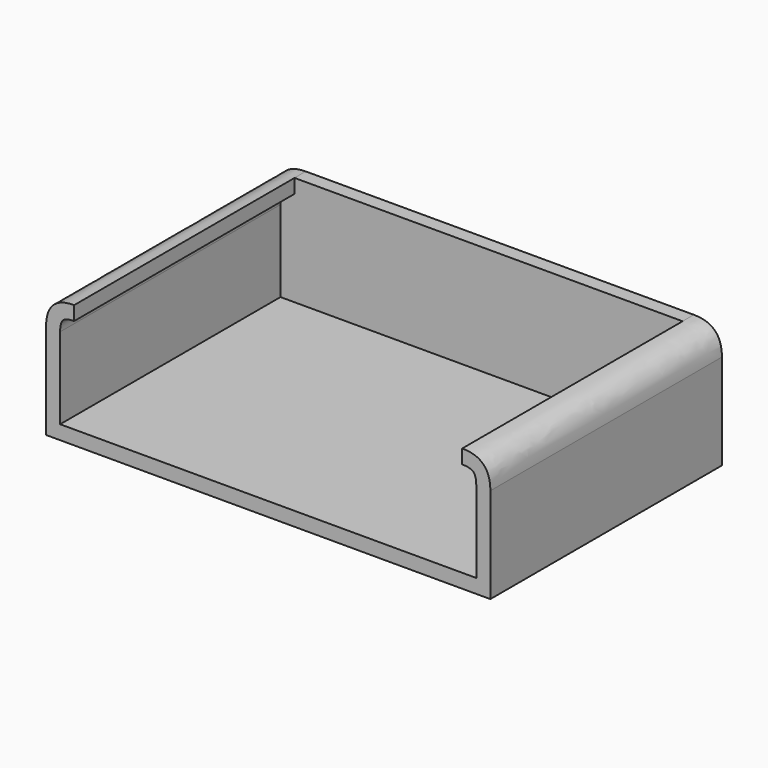
from build123d import *

# Parameters (mm, degrees)
F0_W        = 79.0347680449
F0_H        = 51.5021067113
F1_DEPTH    = 21.9734124839
F2_T1_DEPTH = 76.5021067113
F3_T        = 2.5


# Not quite as in the source:
# - a fillet or chamfer that OpenCascade refuses, or shapes differently, is made with other operations: its cross-section is extruded or revolved along the edge and cut away or added
# - a shell that OpenCascade refuses in one call is made with other operations: the cavity is built on its own and cut out


with BuildPart() as f1:
    # F0 (on Top) → F1 (new body)
    with BuildSketch(Plane.XY):
        with Locations((-4.2740143836, 13.997332193)):
            Rectangle(F0_W, F0_H)
    extrude(amount=F1_DEPTH)

    # F2: fillet of radius 5 on 2 edges, made by hand

    # F2_s2 → F2_t1 (cut)
    with BuildSketch(Plane.XZ.offset(-52.2483855486)):
        with BuildLine():
            add(Edge.make_bspline(
                [(-43.791398406, 16.9734124839), (-43.791398406, 21.9734124839), (-38.791398406, 21.9734124839)],
                knots=[0, 0, 0, 1, 1, 1], degree=2, weights=[1, 1, 1]))
            Line((-38.791398406, 21.9734124839), (-43.791398406, 21.9734124839))
            Line((-43.791398406, 21.9734124839), (-43.791398406, 16.9734124839))
        make_face()
        with BuildLine():
            add(Edge.make_bspline(
                [(35.2433696389, 16.9734124839), (35.2433696389, 21.9734124839), (30.2433696389, 21.9734124839)],
                knots=[0, 0, 0, 1, 1, 1], degree=2, weights=[1, 1, 1]))
            Line((30.2433696389, 21.9734124839), (35.2433696389, 21.9734124839))
            Line((35.2433696389, 21.9734124839), (35.2433696389, 16.9734124839))
        make_face()
    extrude(amount=F2_T1_DEPTH, mode=Mode.SUBTRACT)

    # F3: shell of thickness 2.5, made by hand


with BuildPart() as f3_core1:
    # F3_t2: copy of F1
    add(f1.part)

    # the walls: a layer under each face that stays
    f3_faces = [f3_core1.faces().sort_by_distance(p)[0] for p in [
        (-43.791398406, 13.997332193, 8.4867062419),
        (-4.2740143836, 13.997332193, 0),
        (-42.541398406, 13.997332193, 20.7234124839),
        (-4.2740143836, 39.7483855486, 10.986706242),
        (35.2433696389, 13.997332193, 8.4867062419),
        (33.9933696389, 13.997332193, 20.7234124839),
    ]]
    thicken(f3_faces, amount=-F3_T, mode=Mode.SUBTRACT)


with BuildPart() as f1_1:
    add(f1.part)

    # what is left inside the walls is the cavity
    f3_cavity = [f3_core1.part.solids().sort_by_distance(p)[0] for p in [
        (-4.274014, 4.580314, 2.525),
    ]]
    add(f3_cavity, mode=Mode.SUBTRACT)


solid = f1_1.part
